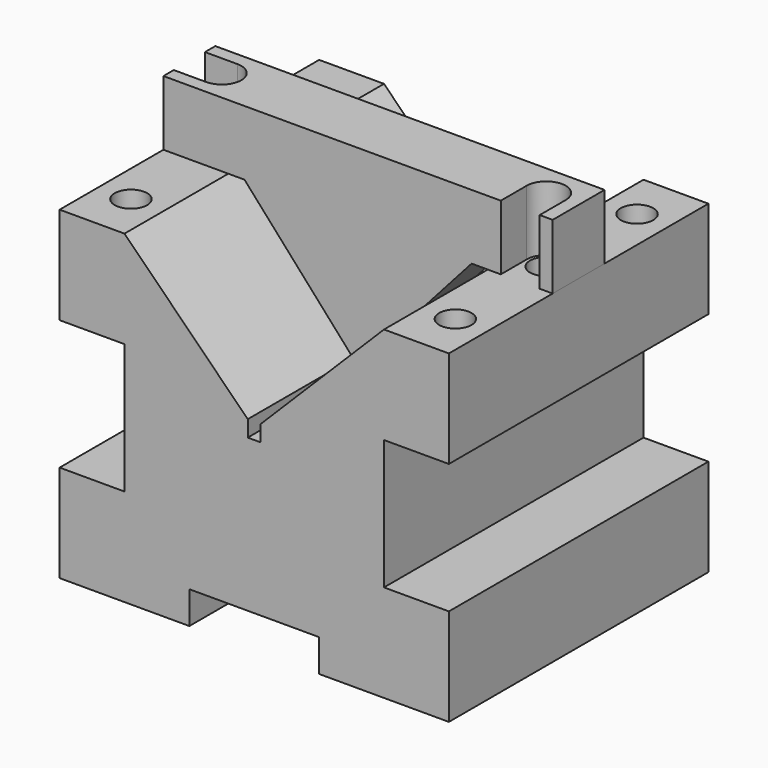
from build123d import *

# Parameters (mm, degrees)
F1_DEPTH = 25
F3_D     = 5
F3_DEPTH = 15
F3_TIP   = 1.5021515476
F4_DEPTH = 5
F6_DEPTH = 60.001


with BuildPart() as f1:
    # F0 (on Front) → F1 (new body, symmetric)
    with BuildSketch(Plane.XZ):
        Polygon((30, 10), (30, 25), (20, 25), (1, 6), (1, 3.5), (-1, 3.5), (-1, 6), (-20, 25), (-30, 25), (-30, 10), (-20, 10), (-20, -10), (-30, -10), (-30, -25), (-10, -25), (-10, -20), (10, -20), (10, -25), (30, -25), (30, -10), (20, -10), (20, 10), align=None)
    extrude(amount=F1_DEPTH, both=True)

    # F3
    with Locations(Plane.XY.offset(25)):
        with Locations((-25, -17.5), (-25, 0), (-25, 17.5), (25, -17.5), (25, 0), (25, 17.5)):
            Hole(F3_D / 2, depth=F3_DEPTH)
            with Locations((0, 0, -(F3_DEPTH + F3_TIP / 2))):  # 118° drill point
                Cone(0, F3_D / 2, F3_TIP, mode=Mode.SUBTRACT)


with BuildPart() as f4:
    # F0 (on Front) → F4 (new body, symmetric)
    with BuildSketch(Plane.XZ):
        Polygon((1, 6.5), (17.5, 25), (-17.5, 25), (-1, 6.5), align=None)
        Polygon((20, 25), (30, 25), (30, 35), (-30, 35), (-30, 25), (-20, 25), (-17.5, 25), (17.5, 25), align=None)
    extrude(amount=F4_DEPTH, both=True)

    # F5 (on face) → F6 (cut, through all)
    with BuildSketch(Plane.XY.offset(35)):
        with BuildLine():
            ThreePointArc((-25, -3), (-22.8786796564, -2.1213203436), (-22, 0))
            ThreePointArc((-22, 0), (-22.8786796564, 2.1213203436), (-25, 3))
            ThreePointArc((-25, 3), (-28, 0), (-25, -3))
        make_face()
        with BuildLine():
            ThreePointArc((-25, -3), (-28, 0), (-25, 3))
            Line((-25, 3), (-30, 3))
            Line((-30, 3), (-30, -3))
            Line((-30, -3), (-25, -3))
        make_face()
        with BuildLine():
            ThreePointArc((28, 0), (25, 3), (22, 0))
            ThreePointArc((22, 0), (25, -3), (28, 0))
        make_face()
        with BuildLine():
            Line((22, 0), (22, -5))
            Line((22, -5), (28, -5))
            Line((28, -5), (28, 0))
            ThreePointArc((28, 0), (25, -3), (22, 0))
        make_face()
    extrude(amount=-F6_DEPTH, mode=Mode.SUBTRACT)


solid = Compound([f1.part, f4.part])
